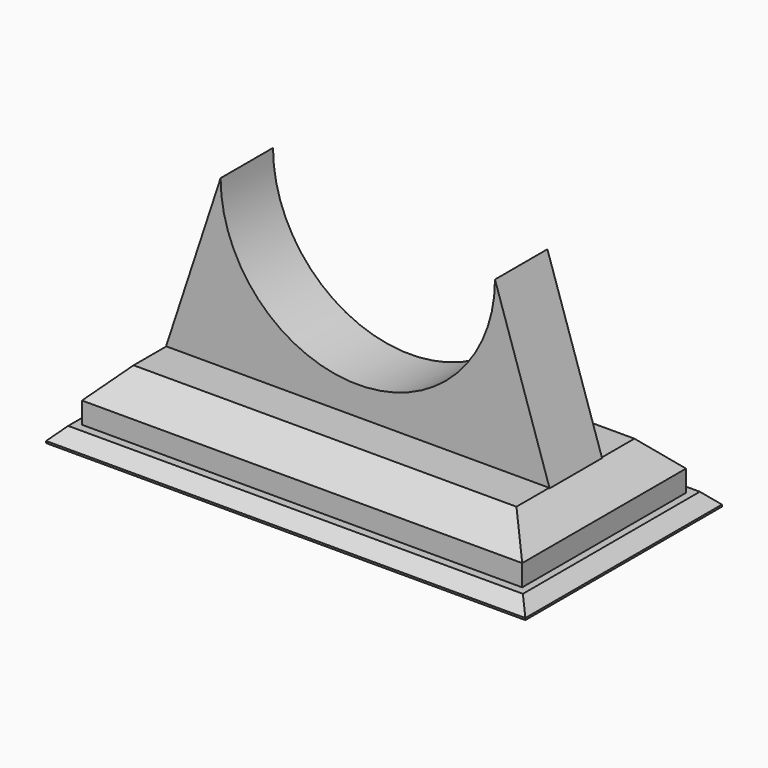
from build123d import *

# Parameters (mm, degrees)
F1_DEPTH     = 10.16
F2_DEPTH     = 31.75
F3_DEPTH     = 38.1
F4_T1_DEPTH  = 182.2402005013
F4_T6_DEPTH  = 109.224523526
F4_T12_DEPTH = 109.224523526
F4_T18_DEPTH = 109.224523526
F4_T25_DEPTH = 109.224523526
F4_T31_DEPTH = 109.224523526
F4_T37_DEPTH = 109.224523526
F4_T43_DEPTH = 109.224523526
F4_T49_DEPTH = 109.224523526
F4_T56_DEPTH = 109.224523526
F4_T62_DEPTH = 109.224523526
F5_SIZE      = 3.81


# Not quite as in the source:
# - a fillet or chamfer that OpenCascade refuses, or shapes differently, is made with other operations: its cross-section is extruded or revolved along the edge and cut away or added


with BuildPart() as f1:
    # F0 (on Front) → F1 (new body, symmetric)
    with BuildSketch(Plane.XZ):
        with BuildLine():
            Line((59.4478547573, -51.4072924852), (42.545, 0))
            ThreePointArc((42.545, 0), (0, -42.545), (-42.545, 0))
            Line((-42.545, 0), (-59.4478547573, -51.4072924852))
            Line((-59.4478547573, -51.4072924852), (0, -51.4072924852))
            Line((0, -51.4072924852), (59.4478547573, -51.4072924852))
        make_face()
    extrude(amount=F1_DEPTH, both=True)

    # F0 (on Front) → F2 (join, symmetric)
    with BuildSketch(Plane.XZ):
        Polygon((0, -51.4072924852), (-59.4478547573, -51.4072924852), (-68.2578384876, -51.4072924852), (-68.2578384876, -66.9220536947), (0, -66.9220536947), align=None)
        Polygon((68.2578384876, -51.4072924852), (59.4478547573, -51.4072924852), (0, -51.4072924852), (0, -66.9220536947), (68.2578384876, -66.9220536947), align=None)
    extrude(amount=F2_DEPTH, both=True)

    # F0 (on Front) → F3 (join, symmetric)
    with BuildSketch(Plane.XZ):
        Polygon((74.3125453591, -66.9220536947), (68.2578384876, -66.9220536947), (0, -66.9220536947), (0, -71.3198781013), (74.3125453591, -71.3198781013), align=None)
        Polygon((0, -71.3198781013), (0, -66.9220536947), (-68.2578384876, -66.9220536947), (-74.3125453591, -66.9220536947), (-74.3125453591, -71.3198781013), align=None)
    extrude(amount=F3_DEPTH, both=True)

    # F4: chamfer of 8.89 on 4 edges, made by hand

    # F4_s2 → F4_t1 (cut)
    with BuildSketch(Plane.YZ.offset(-91.1201002506)):
        Polygon((-31.75, -60.2972924852), (-22.86, -51.4072924852), (-31.75, -51.4072924852), align=None)
        Polygon((31.75, -60.2972924852), (22.86, -51.4072924852), (31.75, -51.4072924852), align=None)
    extrude(amount=F4_T1_DEPTH, mode=Mode.SUBTRACT)


with BuildPart() as f4_tool4:
    # F4_s5 → F4_t6 (new body)
    with BuildSketch(Plane.XZ.offset(54.612261763)):
        Polygon((68.2578384876, -60.2972924852), (59.3678384876, -51.4072924852), (68.2578384876, -51.4072924852), align=None)
    extrude(amount=-F4_T6_DEPTH)

    split(bisect_by=Plane(origin=(38.3941614285, 0, 12.624102589), x_dir=(0, 1, 0), z_dir=(0.949966585, 0, 0.3123515446)), keep=Keep.TOP)

    split(bisect_by=Plane.XZ.offset(10.16), keep=Keep.TOP)


with BuildPart() as f1_1:
    add(f1.part)

    # F4_t3: cut F4_tool4
    add(f4_tool4.part, mode=Mode.SUBTRACT)


with BuildPart() as f4_tool10:
    # F4_s11 → F4_t12 (new body)
    with BuildSketch(Plane.XZ.offset(54.612261763)):
        Polygon((68.2578384876, -60.2972924852), (59.3678384876, -51.4072924852), (68.2578384876, -51.4072924852), align=None)
    extrude(amount=-F4_T12_DEPTH)

    split(bisect_by=Plane(origin=(38.3941614285, 0, 12.624102589), x_dir=(0, 1, 0), z_dir=(-0.949966585, 0, -0.3123515446)), keep=Keep.TOP)

    split(bisect_by=Plane.XZ.offset(10.16), keep=Keep.TOP)


with BuildPart() as f1_2:
    add(f1_1.part)

    # F4_t9: cut F4_tool10
    add(f4_tool10.part, mode=Mode.SUBTRACT)


with BuildPart() as f4_tool16:
    # F4_s17 → F4_t18 (new body)
    with BuildSketch(Plane.XZ.offset(54.612261763)):
        Polygon((68.2578384876, -60.2972924852), (59.3678384876, -51.4072924852), (68.2578384876, -51.4072924852), align=None)
    extrude(amount=-F4_T18_DEPTH)

    split(bisect_by=Plane(origin=(38.3941614285, 0, 12.624102589), x_dir=(0, 1, 0), z_dir=(0.949966585, 0, 0.3123515446)), keep=Keep.TOP)

    split(bisect_by=Plane.XZ.offset(-10.16), keep=Keep.TOP)

    split(bisect_by=Plane.XZ.offset(10.16), keep=Keep.BOTTOM)


with BuildPart() as f1_3:
    add(f1_2.part)

    # F4_t15: cut F4_tool16
    add(f4_tool16.part, mode=Mode.SUBTRACT)


with BuildPart() as f4_tool23:
    # F4_s24 → F4_t25 (new body)
    with BuildSketch(Plane.XZ.offset(54.612261763)):
        Polygon((68.2578384876, -60.2972924852), (59.3678384876, -51.4072924852), (68.2578384876, -51.4072924852), align=None)
    extrude(amount=-F4_T25_DEPTH)

    split(bisect_by=Plane(origin=(38.3941614285, 0, 12.624102589), x_dir=(0, 1, 0), z_dir=(0.949966585, 0, 0.3123515446)), keep=Keep.TOP)

    split(bisect_by=Plane.XZ.offset(-10.16), keep=Keep.BOTTOM)


with BuildPart() as f1_4:
    add(f1_3.part)

    # F4_t22: cut F4_tool23
    add(f4_tool23.part, mode=Mode.SUBTRACT)


with BuildPart() as f4_tool29:
    # F4_s30 → F4_t31 (new body)
    with BuildSketch(Plane.XZ.offset(54.612261763)):
        Polygon((68.2578384876, -60.2972924852), (59.3678384876, -51.4072924852), (68.2578384876, -51.4072924852), align=None)
    extrude(amount=-F4_T31_DEPTH)

    split(bisect_by=Plane(origin=(38.3941614285, 0, 12.624102589), x_dir=(0, 1, 0), z_dir=(-0.949966585, 0, -0.3123515446)), keep=Keep.TOP)

    split(bisect_by=Plane.XZ.offset(-10.16), keep=Keep.BOTTOM)


with BuildPart() as f1_5:
    add(f1_4.part)

    # F4_t28: cut F4_tool29
    add(f4_tool29.part, mode=Mode.SUBTRACT)


with BuildPart() as f4_tool35:
    # F4_s36 → F4_t37 (new body)
    with BuildSketch(Plane.XZ.offset(54.612261763)):
        Polygon((-68.2578384876, -60.2972924852), (-59.3678384876, -51.4072924852), (-68.2578384876, -51.4072924852), align=None)
    extrude(amount=-F4_T37_DEPTH)

    split(bisect_by=Plane(origin=(-38.3941614285, 0, 12.624102589), x_dir=(0, 1, 0), z_dir=(-0.949966585, 0, 0.3123515446)), keep=Keep.TOP)

    split(bisect_by=Plane.XZ.offset(10.16), keep=Keep.TOP)


with BuildPart() as f1_6:
    add(f1_5.part)

    # F4_t34: cut F4_tool35
    add(f4_tool35.part, mode=Mode.SUBTRACT)


with BuildPart() as f4_tool41:
    # F4_s42 → F4_t43 (new body)
    with BuildSketch(Plane.XZ.offset(54.612261763)):
        Polygon((-68.2578384876, -60.2972924852), (-59.3678384876, -51.4072924852), (-68.2578384876, -51.4072924852), align=None)
    extrude(amount=-F4_T43_DEPTH)

    split(bisect_by=Plane(origin=(-38.3941614285, 0, 12.624102589), x_dir=(0, 1, 0), z_dir=(0.949966585, 0, -0.3123515446)), keep=Keep.TOP)

    split(bisect_by=Plane.XZ.offset(10.16), keep=Keep.TOP)


with BuildPart() as f1_7:
    add(f1_6.part)

    # F4_t40: cut F4_tool41
    add(f4_tool41.part, mode=Mode.SUBTRACT)


with BuildPart() as f4_tool47:
    # F4_s48 → F4_t49 (new body)
    with BuildSketch(Plane.XZ.offset(54.612261763)):
        Polygon((-68.2578384876, -60.2972924852), (-59.3678384876, -51.4072924852), (-68.2578384876, -51.4072924852), align=None)
    extrude(amount=-F4_T49_DEPTH)

    split(bisect_by=Plane.XZ.offset(-10.16), keep=Keep.TOP)

    split(bisect_by=Plane(origin=(-38.3941614285, 0, 12.624102589), x_dir=(0, 1, 0), z_dir=(-0.949966585, 0, 0.3123515446)), keep=Keep.TOP)

    split(bisect_by=Plane.XZ.offset(10.16), keep=Keep.BOTTOM)


with BuildPart() as f1_8:
    add(f1_7.part)

    # F4_t46: cut F4_tool47
    add(f4_tool47.part, mode=Mode.SUBTRACT)


with BuildPart() as f4_tool54:
    # F4_s55 → F4_t56 (new body)
    with BuildSketch(Plane.XZ.offset(54.612261763)):
        Polygon((-68.2578384876, -60.2972924852), (-59.3678384876, -51.4072924852), (-68.2578384876, -51.4072924852), align=None)
    extrude(amount=-F4_T56_DEPTH)

    split(bisect_by=Plane.XZ.offset(-10.16), keep=Keep.BOTTOM)

    split(bisect_by=Plane(origin=(-38.3941614285, 0, 12.624102589), x_dir=(0, 1, 0), z_dir=(-0.949966585, 0, 0.3123515446)), keep=Keep.TOP)


with BuildPart() as f1_9:
    add(f1_8.part)

    # F4_t53: cut F4_tool54
    add(f4_tool54.part, mode=Mode.SUBTRACT)


with BuildPart() as f4_tool60:
    # F4_s61 → F4_t62 (new body)
    with BuildSketch(Plane.XZ.offset(54.612261763)):
        Polygon((-68.2578384876, -60.2972924852), (-59.3678384876, -51.4072924852), (-68.2578384876, -51.4072924852), align=None)
    extrude(amount=-F4_T62_DEPTH)

    split(bisect_by=Plane.XZ.offset(-10.16), keep=Keep.BOTTOM)

    split(bisect_by=Plane(origin=(-38.3941614285, 0, 12.624102589), x_dir=(0, 1, 0), z_dir=(0.949966585, 0, -0.3123515446)), keep=Keep.TOP)


with BuildPart() as f1_10:
    add(f1_9.part)

    # F4_t59: cut F4_tool60
    add(f4_tool60.part, mode=Mode.SUBTRACT)

    # F5
    f5_edges = [f1_10.edges().sort_by_distance(p)[0] for p in [
        (0, -38.1, -66.922054),
        (-74.312545, 0, -66.922054),
        (74.312545, 0, -66.922054),
        (0, 38.1, -66.922054),
    ]]
    chamfer(f5_edges, length=F5_SIZE)


solid = f1_10.part
